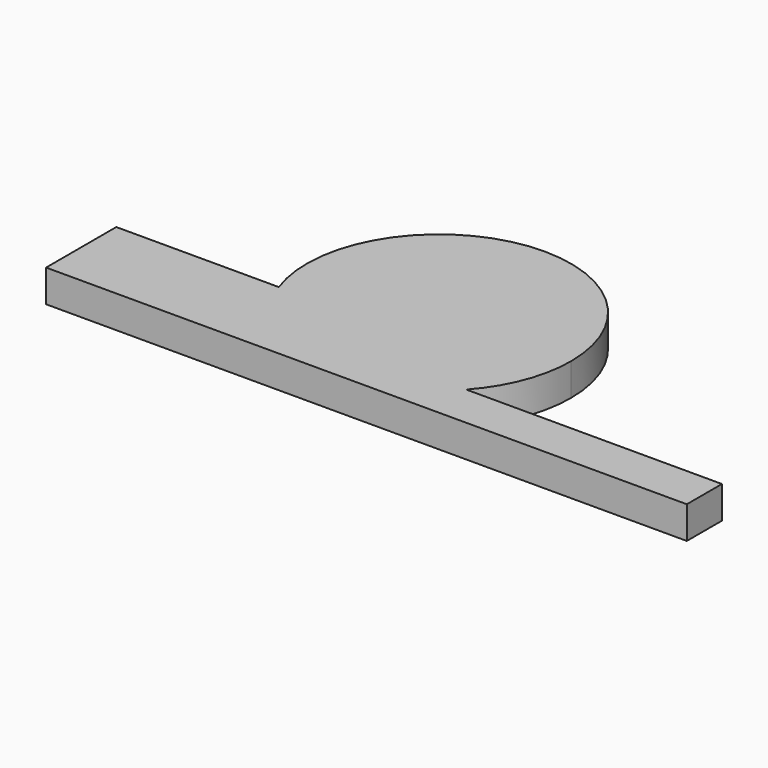
from build123d import *

# Parameters (mm, degrees)
F1_DEPTH = 9.906


# Not quite as in the source:
# - a feature names something its author has since deleted; it is built from what else it names


with BuildPart() as f1:
    # F0 (on Top) → F1 (new body)
    with BuildSketch(Plane.XY):
        with BuildLine():
            Line((-38.1069101836, -13.6540351038), (-87.8979010638, -13.6540351038))
            Line((-87.8979010638, -13.6540351038), (-87.8979010638, -40.5354308852))
            Line((-87.8979010638, -40.5354308852), (20.0543733488, -40.5354308852))
            Line((20.0543733488, -40.5354308852), (20.0543733488, -35.1623575424))
            ThreePointArc((20.0543733488, -35.1623575424), (-14.0401390689, -37.9663505394), (-38.1069101836, -13.6540351038))
        make_face()
        with BuildLine():
            ThreePointArc((30.0739874694, -27.0947329945), (25.3867048086, -31.5291055584), (20.0543733488, -35.1623575424))
            Line((20.0543733488, -35.1623575424), (20.0543733488, -40.5354308852))
            Line((20.0543733488, -40.5354308852), (108.3789337528, -40.5354308852))
            Line((108.3789337528, -40.5354308852), (108.3789337528, -27.0947329945))
            Line((108.3789337528, -27.0947329945), (30.0739874694, -27.0947329945))
        make_face()
        with BuildLine():
            Line((20.0543733488, -13.6540351038), (-38.1069101836, -13.6540351038))
            ThreePointArc((-38.1069101836, -13.6540351038), (-14.0401390689, -37.9663505394), (20.0543733488, -35.1623575424))
            Line((20.0543733488, -35.1623575424), (20.0543733488, -27.0947329945))
            Line((20.0543733488, -27.0947329945), (20.0543733488, -13.6540351038))
        make_face()
        with BuildLine():
            Line((20.0543733488, -27.0947329945), (20.0543733488, -35.1623575424))
            ThreePointArc((20.0543733488, -35.1623575424), (25.3867048086, -31.5291055584), (30.0739874694, -27.0947329945))
            Line((30.0739874694, -27.0947329945), (20.0543733488, -27.0947329945))
        make_face()
        with BuildLine():
            ThreePointArc((40.4792450319, 0), (-6.9292973534, 39.8817516734), (-38.1069101836, -13.6540351038))
            Line((-38.1069101836, -13.6540351038), (20.0543733488, -13.6540351038))
            Line((20.0543733488, -13.6540351038), (20.0543733488, -27.0947329945))
            Line((20.0543733488, -27.0947329945), (30.0739874694, -27.0947329945))
            ThreePointArc((30.0739874694, -27.0947329945), (37.7885008052, -14.5120117574), (40.4792450319, 0))
        make_face()
    extrude(amount=F1_DEPTH)


solid = f1.part
